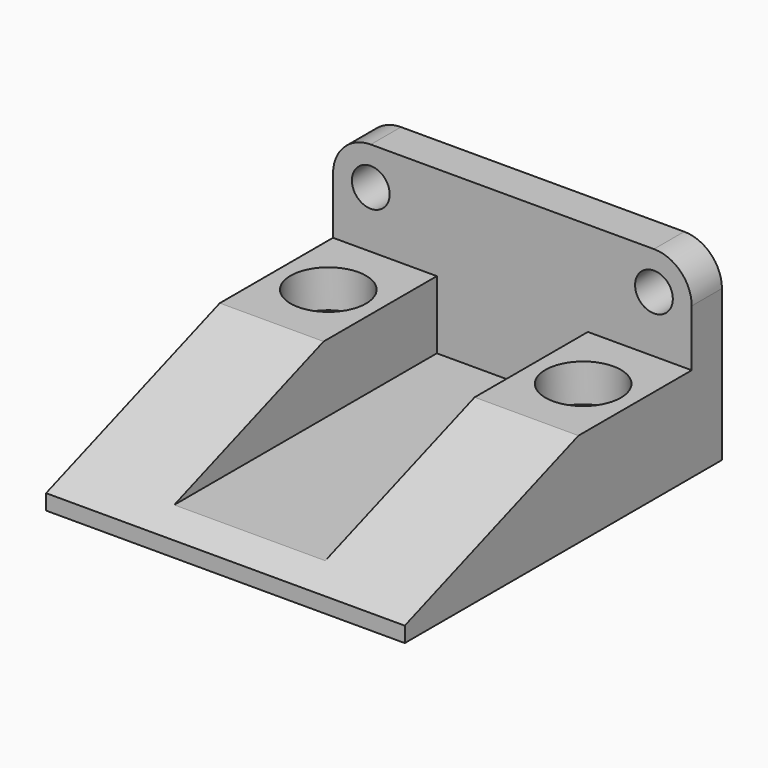
from build123d import *

# Parameters (mm, degrees)
F0_W            = 95
F0_H            = 50
F1_DEPTH        = 10
F2_R            = 10
F3_R            = 5
F4_DEPTH        = 10
F3_W            = 95
F3_H            = 25
F5_DEPTH        = 95
F6_W            = 40
F6_H            = 18
F7_DEPTH        = 95
F8_C1_SIZE2     = 20.9282884703
F8_C1_SIZE      = 57.5
F10_D           = 10
F10_CBORE_D     = 20
F10_CBORE_DEPTH = 10


with BuildPart() as f1:
    # F0 (on Front) → F1 (new body)
    with BuildSketch(Plane.XZ):
        Rectangle(F0_W, F0_H)
    extrude(amount=-F1_DEPTH)

    # F2
    f2_edges = [f1.edges().sort_by_distance(p)[0] for p in [
        (-47.5, 5, 25),
        (47.5, 5, 25),
    ]]
    fillet(f2_edges, radius=F2_R)

    # F3 (on face) → F4 (cut, through all)
    with BuildSketch(Plane.XZ):
        with Locations((-37.5, 15)):
            Circle(F3_R)
        with Locations((37.5, 15)):
            Circle(F3_R)
    extrude(amount=-F4_DEPTH, mode=Mode.SUBTRACT)

    # F3 (on face) → F5 (join)
    with BuildSketch(Plane.XZ):
        with Locations((0, -12.5)):
            Rectangle(F3_W, F3_H)
    extrude(amount=F5_DEPTH)

    # F6 (on face) → F7 (cut, through all)
    with BuildSketch(Plane.XZ.offset(95)):
        with Locations((0, -9)):
            Rectangle(F6_W, F6_H)
        with Locations((0, 9)):
            Rectangle(F6_W, F6_H)
    extrude(amount=-F7_DEPTH, mode=Mode.SUBTRACT)

    # F8: chamfer of 57.5 x 20.9282884703 on 2 edges, made by hand

    # F8_c1
    f8_c1_edges = [f1.edges().sort_by_distance(p)[0] for p in [
        (33.75, -95, 0),
    ]]
    f8_c1_side = f1.faces().sort_by_distance((33.75, -94.5814342306, 0))[0]
    chamfer(f8_c1_edges, length=F8_C1_SIZE, length2=F8_C1_SIZE2, reference=f8_c1_side)

    # F10 (through all)
    with Locations(Plane.XY):
        with Locations((-33.75, -18.75), (33.75, -18.75)):
            CounterBoreHole(F10_D / 2, F10_CBORE_D / 2, F10_CBORE_DEPTH)


solid = f1.part
